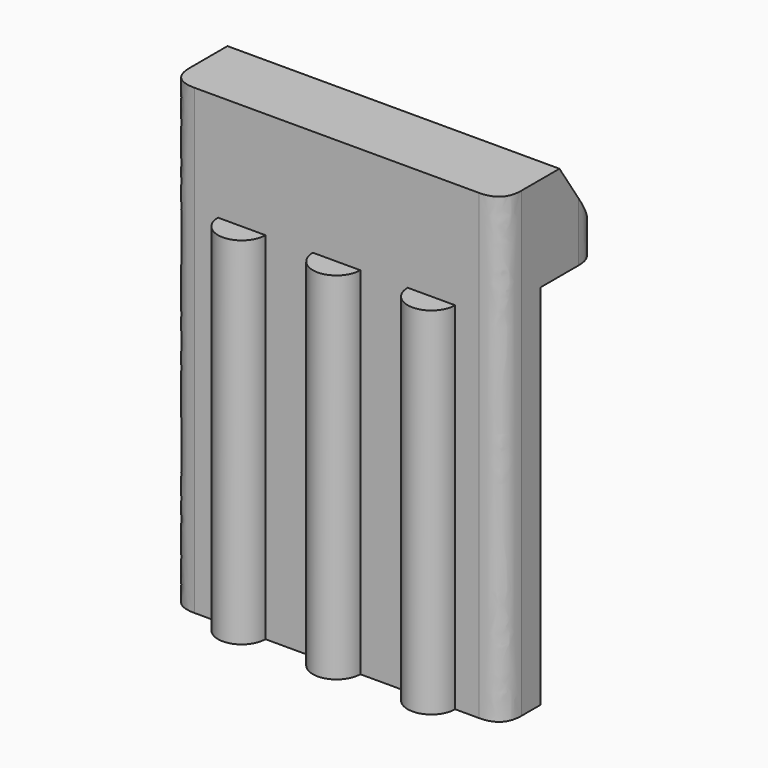
from build123d import *

# Parameters (mm, degrees)
F0_W        = 14
F0_H        = 2
F1_DEPTH    = 15.5
F2_W        = 14
F2_H        = 3
F2_H_2      = 2
F3_DEPTH    = 4
F4_SIZE2    = 2
F4_SIZE     = 3
F5_T1_DEPTH = 24.5
F5_T3_DEPTH = 6
F7_DEPTH    = 15


# Not quite as in the source:
# - a fillet or chamfer that OpenCascade refuses, or shapes differently, is made with other operations: its cross-section is extruded or revolved along the edge and cut away or added


with BuildPart() as f1:
    # F0 (on Top) → F1 (new body)
    with BuildSketch(Plane.XY):
        Rectangle(F0_W, F0_H)
    extrude(amount=F1_DEPTH)

    # F2 (on face) → F3 (join)
    with BuildSketch(Plane.XY.offset(15.5)):
        with Locations((0, 2.5)):
            Rectangle(F2_W, F2_H)
        Rectangle(F2_W, F2_H_2)
    extrude(amount=F3_DEPTH)

    # F4
    f4_edges = [f1.edges().sort_by_distance(p)[0] for p in [
        (0, 4, 19.5),
    ]]
    f4_side = f1.faces().sort_by_distance((0, 4, 17.5))[0]
    chamfer(f4_edges, length=F4_SIZE, length2=F4_SIZE2, reference=f4_side)

    # F5: fillet of radius 1 on 4 edges, made by hand

    # F5_s2 → F5_t1 (cut)
    with BuildSketch(Plane.XY.offset(-2.5)):
        with BuildLine():
            add(Edge.make_bspline(
                [(-7, 0), (-7, -1), (-6, -1)],
                knots=[0, 0, 0, 1, 1, 1], degree=2, weights=[1, 1, 1]))
            Line((-6, -1), (-7, -1))
            Line((-7, -1), (-7, 0))
        make_face()
        with BuildLine():
            add(Edge.make_bspline(
                [(7, 0), (7, -1), (6, -1)],
                knots=[0, 0, 0, 1, 1, 1], degree=2, weights=[1, 1, 1]))
            Line((6, -1), (7, -1))
            Line((7, -1), (7, 0))
        make_face()
    extrude(amount=F5_T1_DEPTH, mode=Mode.SUBTRACT)

    # F5_s4 → F5_t3 (cut)
    with BuildSketch(Plane.XY.offset(13)):
        with BuildLine():
            add(Edge.make_bspline(
                [(-6, 4), (-7, 4), (-7, 3)],
                knots=[0, 0, 0, 1, 1, 1], degree=2, weights=[1, 1, 1]))
            Line((-7, 3), (-7, 4))
            Line((-7, 4), (-6, 4))
        make_face()
        with BuildLine():
            add(Edge.make_bspline(
                [(6, 4), (7, 4), (7, 3)],
                knots=[0, 0, 0, 1, 1, 1], degree=2, weights=[1, 1, 1]))
            Line((7, 3), (7, 4))
            Line((7, 4), (6, 4))
        make_face()
    extrude(amount=F5_T3_DEPTH, mode=Mode.SUBTRACT)

    # F6 (on face) → F7 (join)
    with BuildSketch(Plane(origin=(0, 0, 0), x_dir=(1, 0, 0), z_dir=(0, 0, -1))):
        with BuildLine():
            Line((-1, 1), (1, 1))
            ThreePointArc((1, 1), (0, 2), (-1, 1))
        make_face()
        with BuildLine():
            Line((5, 1), (3, 1))
            ThreePointArc((3, 1), (4, 0), (5, 1))
        make_face()
        with BuildLine():
            ThreePointArc((5, 1), (4, 2), (3, 1))
            Line((3, 1), (5, 1))
        make_face()
        with BuildLine():
            Line((-5, 1), (-3, 1))
            ThreePointArc((-3, 1), (-4, 2), (-5, 1))
        make_face()
    extrude(amount=-F7_DEPTH)


solid = f1.part
